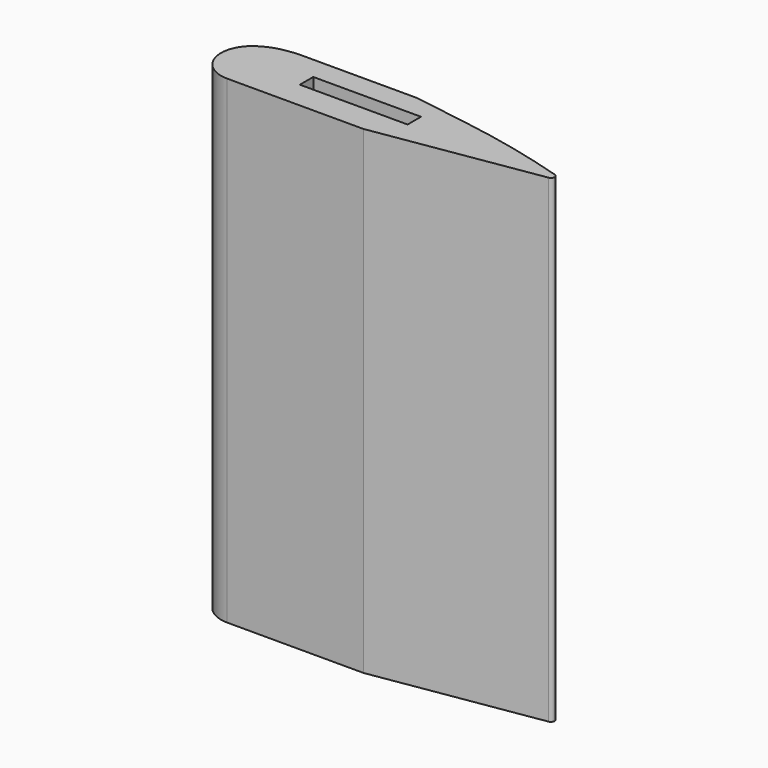
from build123d import *

# Parameters (mm, degrees)
F0_W        = 75.0949196517
F0_H        = 14.2217068933
F0_W_2      = 22.86
F0_H_2      = 3.556
F1_DEPTH    = 101.6
F2_T1_DEPTH = 165.9870757085
F3_R        = 6.5531023684
F4_SIZE2    = 6.0344471764
F4_SIZE     = 38.1
F4_2_SIZE2  = 6.0344471764
F4_2_SIZE   = 38.1
F5_T1_DEPTH = 234.6078157438
F6_T1_DEPTH = 118.09821105


# Not quite as in the source:
# - a fillet or chamfer that OpenCascade refuses, or shapes differently, is made with other operations: its cross-section is extruded or revolved along the edge and cut away or added


with BuildPart() as f1:
    # F0 (on Top) → F1 (new body)
    with BuildSketch(Plane.XY):
        with Locations((7.2930697352, -0.4826590884)):
            Rectangle(F0_W, F0_H)
        Rectangle(F0_W_2, F0_H_2, mode=Mode.SUBTRACT)
    extrude(amount=F1_DEPTH)

    # F2: fillet of radius 12.8774151417 on 1 edges, made by hand

    # F2_s2 → F2_t1 (cut)
    with BuildSketch(Plane.XY.offset(-32.1935378542)):
        with BuildLine():
            add(Edge.make_bspline(
                [(-17.376974949, 6.6281943582), (-30.2543900907, 6.6281943582), (-30.2543900907, -6.2492207835)],
                knots=[0, 0, 0, 1, 1, 1], degree=2, weights=[1, 1, 1]))
            Line((-30.2543900907, -6.2492207835), (-30.2543900907, 6.6281943582))
            Line((-30.2543900907, 6.6281943582), (-17.376974949, 6.6281943582))
        make_face()
    extrude(amount=F2_T1_DEPTH, mode=Mode.SUBTRACT)

    # F3
    f3_edges = [f1.edges().sort_by_distance(p)[0] for p in [
        (-30.25439, -7.593513, 50.8),
    ]]
    fillet(f3_edges, radius=F3_R)

    # F4
    f4_edges = [f1.edges().sort_by_distance(p)[0] for p in [
        (44.84053, 6.628194, 50.8),
    ]]
    f4_side = f1.faces().sort_by_distance((13.731777, 6.628194, 50.8))[0]
    chamfer(f4_edges, length=F4_SIZE, length2=F4_SIZE2, reference=f4_side)

    # F4#2
    f4_2_edges = [f1.edges().sort_by_distance(p)[0] for p in [
        (44.84053, -7.593513, 50.8),
    ]]
    f4_2_side = f1.faces().sort_by_distance((11.322316, -7.593513, 50.8))[0]
    chamfer(f4_2_edges, length=F4_2_SIZE, length2=F4_2_SIZE2, reference=f4_2_side)

    # F5: fillet of radius 171.7049577379 on 1 edges, made by hand

    # F5_s2 → F5_t1 (cut)
    with BuildSketch(Plane.XY.offset(-66.5039078719)):
        with BuildLine():
            ThreePointArc((44.840529561, -1.5590653587), (31.8279082353, 2.1157050987), (18.5664757974, 4.7551484822))
            Line((18.5664757974, 4.7551484822), (44.840529561, 0.5937471818))
            Line((44.840529561, 0.5937471818), (44.840529561, -1.5590653587))
        make_face()
    extrude(amount=F5_T1_DEPTH, mode=Mode.SUBTRACT)

    # F6: fillet of radius 0.7744916247 on 1 edges, made by hand

    # F6_s2 → F6_t1 (cut)
    with BuildSketch(Plane.XY.offset(-8.249105525)):
        with BuildLine():
            ThreePointArc((41.5888697855, -2.0740776724), (42.240352702, -1.3626428472), (41.6931850181, -0.5681763427))
            ThreePointArc((41.6931850181, -0.5681763427), (43.2692375752, -1.0560603886), (44.840529561, -1.5590653587))
            Line((44.840529561, -1.5590653587), (41.5888697855, -2.0740776724))
        make_face()
    extrude(amount=F6_T1_DEPTH, mode=Mode.SUBTRACT)


solid = f1.part
